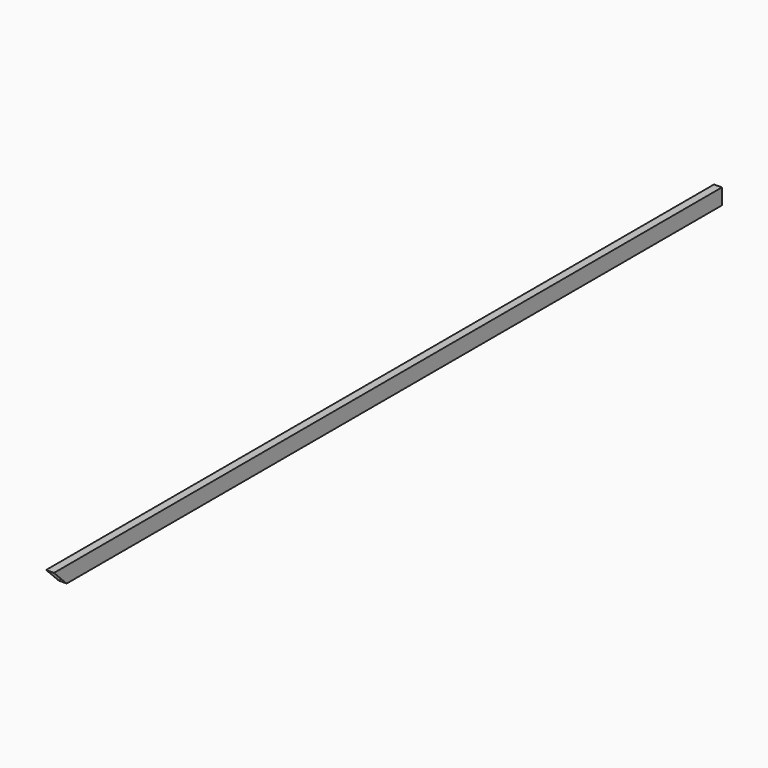
from build123d import *

# Parameters (mm, degrees)
F0_W        = 50
F0_H        = 100
F0_W_2      = 44
F0_H_2      = 94
F1_DEPTH    = 5270
F2_T1_DEPTH = 564.3365975932


# Not quite as in the source:
# - a fillet or chamfer that OpenCascade refuses, or shapes differently, is made with other operations: its cross-section is extruded or revolved along the edge and cut away or added


with BuildPart() as f1:
    # F0 (on Front) → F1 (new body)
    with BuildSketch(Plane.XZ):
        with Locations((-9.287606366, 17.9927872233)):
            Rectangle(F0_W, F0_H)
        with Locations((-9.287606366, 17.9927872233)):
            Rectangle(F0_W_2, F0_H_2, mode=Mode.SUBTRACT)
    extrude(amount=F1_DEPTH)

    # F2: chamfer of 100 on 1 edges, made by hand

    # F2_s2 → F2_t1 (cut)
    with BuildSketch(Plane.YZ.offset(-291.4559051626)):
        Polygon((-5170, -32.0072127767), (-5270, 67.9927872233), (-5270, -32.0072127767), align=None)
    extrude(amount=F2_T1_DEPTH, mode=Mode.SUBTRACT)


solid = f1.part
